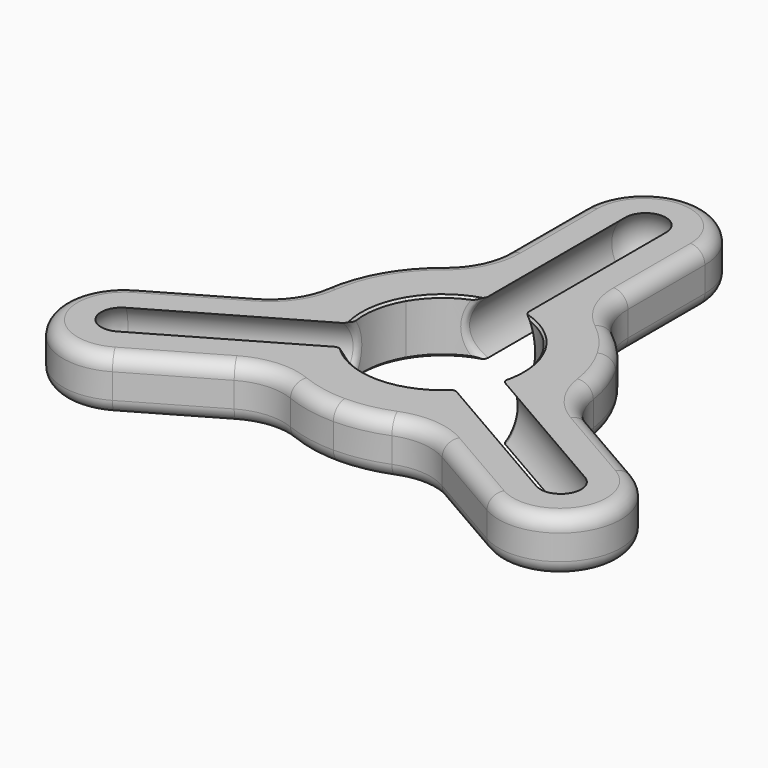
from build123d import *

# Parameters (mm, degrees)
F1_DEPTH      = 3.75
F1_DEPTH_BACK = 3.75
F2_R          = 4.7
F3_DEPTH      = 40
F4_R          = 4.7
F5_R          = 8.5
F7_T2_ANGLE   = 53.1118954737
F7_T4_ANGLE   = 53.1118954737
F7_T6_ANGLE   = 53.1118954737
F7_T8_ANGLE   = 53.1118954737
F8_R          = 1
F10_COUNT     = 3
F11_R         = 2


# Not quite as in the source:
# - a fillet or chamfer that OpenCascade refuses, or shapes differently, is made with other operations: its cross-section is extruded or revolved along the edge and cut away or added


with BuildPart() as f1:
    # F0 (on Top) → F1 (new body, two sides)
    with BuildSketch(Plane.XY) as f1_sk:
        with BuildLine():
            ThreePointArc((-9.5262794416, 5.5), (0, 11), (9.5262794416, 5.5))
            Line((9.5262794416, 5.5), (16.4544826719, 9.5))
            ThreePointArc((16.4544826719, 9.5), (13.0275279843, 13.8305283564), (8.5, 16.992645468))
            Line((8.5, 16.992645468), (8.5, 35))
            ThreePointArc((8.5, 35), (0, 43.5), (-8.5, 35))
            Line((-8.5, 35), (-8.5, 16.992645468))
            ThreePointArc((-8.5, 16.992645468), (-13.0275279843, 13.8305283564), (-16.4544826719, 9.5))
            Line((-16.4544826719, 9.5), (-9.5262794416, 5.5))
        make_face()
    extrude(amount=F1_DEPTH)
    extrude(f1_sk.sketch, amount=-F1_DEPTH_BACK)

    # F5
    f5_edges = [f1.edges().sort_by_distance(p)[0] for p in [
        (-8.5, 16.992645, 0),
        (8.5, 16.992645, 0),
    ]]
    fillet(f5_edges, radius=F5_R)


with BuildPart() as f3:
    # F2 (on Front) → F3 (new body)
    with BuildSketch(Plane.XZ):
        Circle(F2_R)
    extrude(amount=-F3_DEPTH)

    # F4
    f4_edges = [f3.edges().sort_by_distance(p)[0] for p in [
        (-4.7, 40, 0),
    ]]
    fillet(f4_edges, radius=F4_R)


with BuildPart() as f1_1:
    add(f1.part)

    # F6: cut F3
    add(f3.part, mode=Mode.SUBTRACT)

    # F7: chamfer of 0.3 on 4 edges, made by hand

    # F7_s1 → F7_t2 (revolve, cut)
    with BuildSketch(Plane(origin=(0, 0, 0), x_dir=(0, 0, 1), z_dir=(-0.438073888, -0.8989389682, 0))):
        Polygon((3.75, 11.3), (3.45, 11), (3.75, 11), align=None)
    revolve(axis=Axis((0, 0, 3.75), (0, 0, -1)), revolution_arc=F7_T2_ANGLE, mode=Mode.SUBTRACT)

    # F7_s3 → F7_t4 (revolve, cut)
    with BuildSketch(Plane(origin=(0, 0, 0), x_dir=(0, 0, 1), z_dir=(-0.438073888, -0.8989389682, 0))):
        Polygon((-3.75, 11.3), (-3.45, 11), (-3.75, 11), align=None)
    revolve(axis=Axis((0, 0, -3.75), (0, 0, -1)), revolution_arc=F7_T4_ANGLE, mode=Mode.SUBTRACT)

    # F7_s5 → F7_t6 (revolve, cut)
    with BuildSketch(Plane(origin=(0, 0, 0), x_dir=(0, 0, 1), z_dir=(-0.9819354297, 0.1892163097, 0))):
        Polygon((-3.75, 11.3), (-3.45, 11), (-3.75, 11), align=None)
    revolve(axis=Axis((0, 0, -3.75), (0, 0, -1)), revolution_arc=F7_T6_ANGLE, mode=Mode.SUBTRACT)

    # F7_s7 → F7_t8 (revolve, cut)
    with BuildSketch(Plane(origin=(0, 0, 0), x_dir=(0, 0, 1), z_dir=(-0.9819354297, 0.1892163097, 0))):
        Polygon((3.75, 11.3), (3.45, 11), (3.75, 11), align=None)
    revolve(axis=Axis((0, 0, 3.75), (0, 0, -1)), revolution_arc=F7_T8_ANGLE, mode=Mode.SUBTRACT)

    # F8
    f8_edges = [f1_1.edges().sort_by_distance(p)[0] for p in [
        (-4.7, 9.945351, 0),
        (4.7, 9.945351, 0),
    ]]
    fillet(f8_edges, radius=F8_R)

    # F10: F1 ×3 about axis
    f10_axis = Axis((0, 0, 12.4659836292), (0, 0, 1))


with BuildPart() as f1_2:
    add(f1_1.part)
    for i in range(1, F10_COUNT):
        add(f1_1.part.rotate(f10_axis, i * 360 / F10_COUNT))

    # F11
    f11_edges = [f1_2.edges().sort_by_distance(p)[0] for p in [
        (-8.5, 28.307983, 3.75),
        (-20.265433, -21.515208, -3.75),
    ]]
    fillet(f11_edges, radius=F11_R)


solid = f1_2.part
